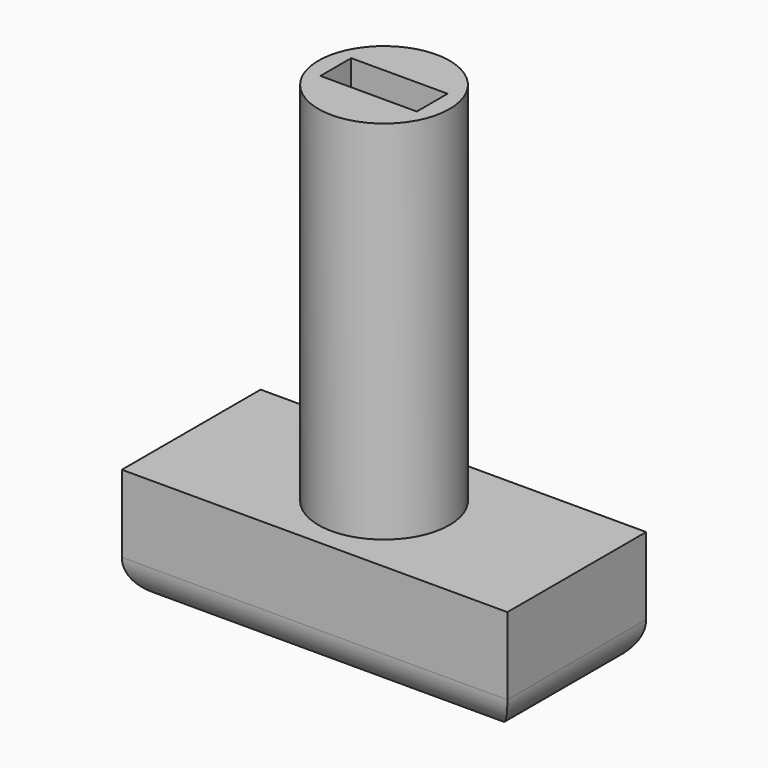
from build123d import *

# Parameters (mm, degrees)
F0_R     = 4.318
F0_W     = 6.35
F0_H     = 2.54
F1_DEPTH = 24.13
F2_W     = 25.4
F2_H     = 11.43
F2_R     = 4.318
F2_W_2   = 6.35
F2_H_2   = 2.54
F3_DEPTH = 7.62
F4_R     = 2.54


with BuildPart() as f1:
    # F0 (on Top) → F1 (new body)
    with BuildSketch(Plane.XY):
        Circle(F0_R)
        Rectangle(F0_W, F0_H, mode=Mode.SUBTRACT)
    extrude(amount=F1_DEPTH)

    # F2 (on face) → F3 (join)
    with BuildSketch(Plane(origin=(0, 0, 0), x_dir=(1, 0, 0), z_dir=(0, 0, -1))):
        Rectangle(F2_W, F2_H)
        Circle(F2_R, mode=Mode.SUBTRACT)
        Circle(F2_R)
        Rectangle(F2_W_2, F2_H_2, mode=Mode.SUBTRACT)
        Rectangle(F2_W_2, F2_H_2)
    extrude(amount=F3_DEPTH)

    # F4
    f4_edges = [f1.edges().sort_by_distance(p)[0] for p in [
        (12.7, 0, -7.62),
        (0, -5.715, -7.62),
        (-12.7, 0, -7.62),
        (0, 5.715, -7.62),
    ]]
    fillet(f4_edges, radius=F4_R)


solid = f1.part
